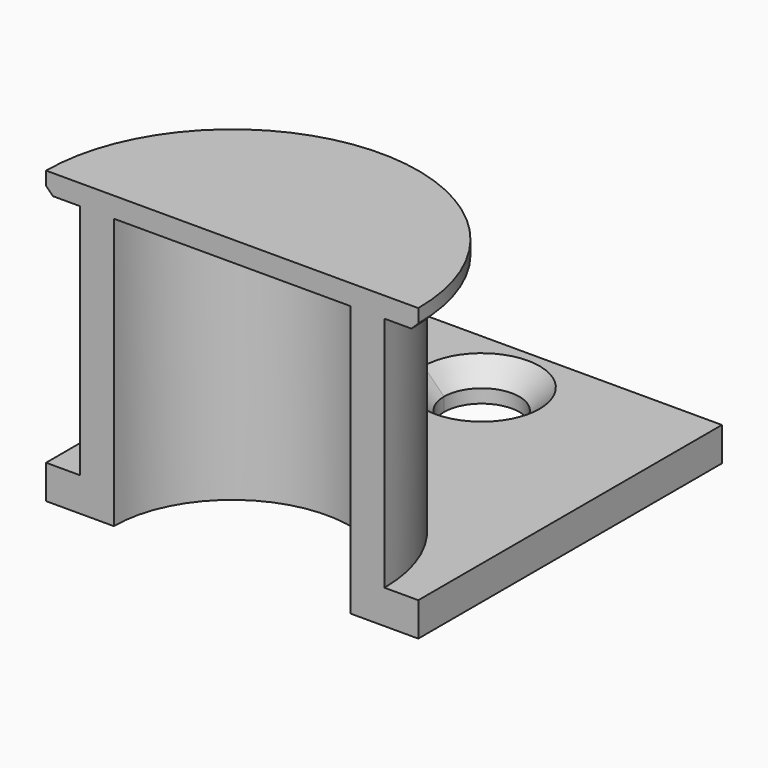
from build123d import *

# Parameters (mm, degrees)
F1_DEPTH = 5
F2_DEPTH = 40
F3_SIZE  = 3
F5_DEPTH = 3
F6_SIZE  = 1


with BuildPart() as f1:
    # F0 (on Top) → F1 (new body)
    with BuildSketch(Plane.XY):
        with BuildLine():
            Line((55, 56.0835413635), (0, 56.0835413635))
            Line((0, 56.0835413635), (0, 46.0835413635))
            Line((0, 46.0835413635), (21.9390119762, 46.0835413635))
            ThreePointArc((21.9390119762, 46.0835413635), (27.5, 51.6445293873), (33.0609880238, 46.0835413635))
            Line((33.0609880238, 46.0835413635), (55, 46.0835413635))
            Line((55, 46.0835413635), (55, 56.0835413635))
        make_face()
        with BuildLine():
            Line((21.9390119762, 46.0835413635), (0, 46.0835413635))
            Line((0, 46.0835413635), (0, 0))
            Line((0, 0), (5, 0))
            ThreePointArc((5, 0), (27.5, 22.5), (50, 0))
            Line((50, 0), (55, 0))
            Line((55, 0), (55, 46.0835413635))
            Line((55, 46.0835413635), (33.0609880238, 46.0835413635))
            ThreePointArc((33.0609880238, 46.0835413635), (27.5, 40.5225533396), (21.9390119762, 46.0835413635))
        make_face()
    extrude(amount=F1_DEPTH)

    # F0 (on Top) → F2 (join)
    with BuildSketch(Plane.XY):
        with BuildLine():
            ThreePointArc((50, 0), (27.5, 22.5), (5, 0))
            Line((5, 0), (10, 0))
            ThreePointArc((10, 0), (27.5, 17.5), (45, 0))
            Line((45, 0), (50, 0))
        make_face()
    extrude(amount=F2_DEPTH)

    # F3
    f3_edges = [f1.edges().sort_by_distance(p)[0] for p in [
        (21.939012, 46.083541, 5),
    ]]
    chamfer(f3_edges, length=F3_SIZE)

    # F4 (on face) → F5 (join)
    with BuildSketch(Plane.XY.offset(40)):
        with BuildLine():
            Line((50, 0), (55, 0))
            ThreePointArc((55, 0), (27.5, 27.5), (0, 0))
            Line((0, 0), (5, 0))
            ThreePointArc((5, 0), (27.5, 22.5), (50, 0))
        make_face()
        with BuildLine():
            Line((45, 0), (50, 0))
            ThreePointArc((50, 0), (27.5, 22.5), (5, 0))
            Line((5, 0), (10, 0))
            ThreePointArc((10, 0), (27.5, 17.5), (45, 0))
        make_face()
        with BuildLine():
            Line((10, 0), (45, 0))
            ThreePointArc((45, 0), (27.5, 17.5), (10, 0))
        make_face()
    extrude(amount=F5_DEPTH)

    # F6
    f6_edges = [f1.edges().sort_by_distance(p)[0] for p in [
        (27.5, 27.5, 40),
    ]]
    chamfer(f6_edges, length=F6_SIZE)


solid = f1.part
